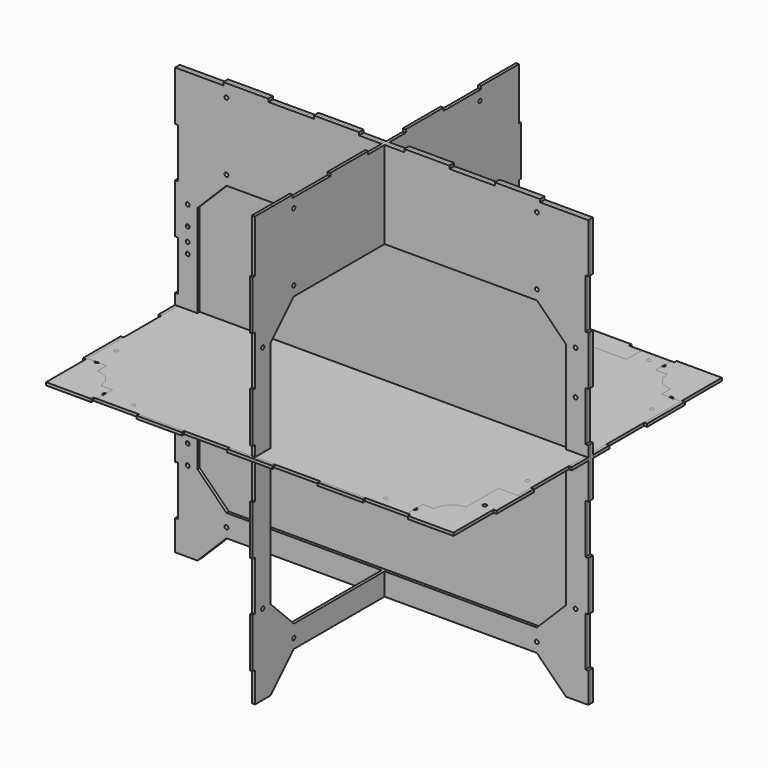
from build123d import *

# Parameters (mm, degrees)
F1_R     = 2
F2_DEPTH = 3
F3_R     = 2
F4_DEPTH = 3
F5_DEPTH = 3
F6_R     = 2
F7_DEPTH = 3
F8_R     = 2
F9_DEPTH = 3


# Not quite as in the source:
# - a feature names something its author has since deleted; it is built from what else it names


with BuildPart() as f2:
    # F1 (on Top) → F2 (new body)
    with BuildSketch(Plane.XY):
        Polygon((163.3333333333, -173), (210, -173), (210, -170), (210, -121.4285714286), (213, -121.4285714286), (213, -72.8571428571), (210, -72.8571428571), (210, -24.2857142857), (213, -24.2857142857), (213, 24.2857142857), (210, 24.2857142857), (210, 72.8571428571), (213, 72.8571428571), (213, 121.4285714286), (210, 121.4285714286), (210, 170), (210, 173), (163.3333333333, 173), (163.3333333333, 170), (116.6666666667, 170), (116.6666666667, 173), (70, 173), (70, 170), (23.3333333333, 170), (23.3333333333, 173), (-23.3333333333, 173), (-23.3333333333, 170), (-70, 170), (-70, 173), (-116.6666666667, 173), (-116.6666666667, 170), (-163.3333333333, 170), (-163.3333333333, 173), (-210, 173), (-210, 170), (-210, 121.4285714286), (-213, 121.4285714286), (-213, 72.8571428571), (-210, 72.8571428571), (-210, 24.2857142857), (-213, 24.2857142857), (-213, -24.2857142857), (-210, -24.2857142857), (-210, -72.8571428571), (-213, -72.8571428571), (-213, -121.4285714286), (-210, -121.4285714286), (-210, -170), (-210, -173), (-163.3333333333, -173), (-163.3333333333, -170), (-116.6666666667, -170), (-116.6666666667, -173), (-70, -173), (-70, -170), (-23.3333333333, -170), (-23.3333333333, -173), (23.3333333333, -173), (23.3333333333, -170), (70, -170), (70, -173), (116.6666666667, -173), (116.6666666667, -170), (163.3333333333, -170), align=None)
        with Locations((-160, -160)):
            Circle(F1_R, mode=Mode.SUBTRACT)
        with Locations((-200, -120)):
            Circle(F1_R, mode=Mode.SUBTRACT)
        with Locations((160, -160)):
            Circle(F1_R, mode=Mode.SUBTRACT)
        with Locations((200, -120)):
            Circle(F1_R, mode=Mode.SUBTRACT)
        with Locations((-200, 120)):
            Circle(F1_R, mode=Mode.SUBTRACT)
        with Locations((-160, 160)):
            Circle(F1_R, mode=Mode.SUBTRACT)
        Polygon((190, -120), (160, -150), (-160, -150), (-190, -120), (-190, 120), (-160, 150), (160, 150), (190, 120), align=None, mode=Mode.SUBTRACT)
        with Locations((200, 120)):
            Circle(F1_R, mode=Mode.SUBTRACT)
        with Locations((160, 160)):
            Circle(F1_R, mode=Mode.SUBTRACT)
    extrude(amount=F2_DEPTH)


with BuildPart() as f4:
    # F3 (on Front) → F4 (new body)
    with BuildSketch(Plane.XZ):
        Polygon((190, -221.5), (213, -221.5), (213, -190.3888888889), (210, -190.3888888889), (210, -139.2777777778), (213, -139.2777777778), (213, -88.1666666667), (210, -88.1666666667), (210, -37.0555555556), (213, -37.0555555556), (213, 14.0555555556), (210, 14.0555555556), (210, 65.1666666667), (213, 65.1666666667), (213, 116.2777777778), (210, 116.2777777778), (210, 167.3888888889), (213, 167.3888888889), (213, 218.5), (210, 218.5), (163.3333333333, 218.5), (163.3333333333, 221.5), (116.6666666667, 221.5), (116.6666666667, 218.5), (70, 218.5), (70, 221.5), (23.3333333333, 221.5), (23.3333333333, 218.5), (-23.3333333333, 218.5), (-23.3333333333, 221.5), (-70, 221.5), (-70, 218.5), (-116.6666666667, 218.5), (-116.6666666667, 221.5), (-163.3333333333, 221.5), (-163.3333333333, 218.5), (-210, 218.5), (-213, 218.5), (-213, 167.3888888889), (-210, 167.3888888889), (-210, 116.2777777778), (-213, 116.2777777778), (-213, 65.1666666667), (-210, 65.1666666667), (-210, 14.0555555556), (-213, 14.0555555556), (-213, -37.0555555556), (-210, -37.0555555556), (-210, -88.1666666667), (-213, -88.1666666667), (-213, -139.2777777778), (-210, -139.2777777778), (-210, -190.3888888889), (-213, -190.3888888889), (-213, -221.5), (-190, -221.5), (-160, -191.5), (160, -191.5), align=None)
        with Locations((-160, -181.5)):
            Circle(F3_R, mode=Mode.SUBTRACT)
        with Locations((-200, -138.5)):
            Circle(F3_R, mode=Mode.SUBTRACT)
        with Locations((-200, -118.5)):
            Circle(F3_R, mode=Mode.SUBTRACT)
        with Locations((-200, -104.5)):
            Circle(F3_R, mode=Mode.SUBTRACT)
        with Locations((160, -181.5)):
            Circle(F3_R, mode=Mode.SUBTRACT)
        with Locations((200, -138.5)):
            Circle(F3_R, mode=Mode.SUBTRACT)
        Polygon((-160, 128.5), (160, 128.5), (190, 98.5), (190, -138.5), (160, -168.5), (-160, -168.5), (-190, -138.5), (-190, 98.5), align=None, mode=Mode.SUBTRACT)
        with Locations((-200, 53.5)):
            Circle(F3_R, mode=Mode.SUBTRACT)
        with Locations((-200, 64.5)):
            Circle(F3_R, mode=Mode.SUBTRACT)
        with Locations((-200, 78.5)):
            Circle(F3_R, mode=Mode.SUBTRACT)
        with Locations((-200, 98.5)):
            Circle(F3_R, mode=Mode.SUBTRACT)
        with Locations((-160, 138.5)):
            Circle(F3_R, mode=Mode.SUBTRACT)
        with Locations((-160, 208.5)):
            Circle(F3_R, mode=Mode.SUBTRACT)
        with Locations((-140, 208.5)):
            Circle(F3_R, mode=Mode.SUBTRACT)
        with Locations((-126, 208.5)):
            Circle(F3_R, mode=Mode.SUBTRACT)
        with Locations((200, 53.5)):
            Circle(F3_R, mode=Mode.SUBTRACT)
        with Locations((200, 98.5)):
            Circle(F3_R, mode=Mode.SUBTRACT)
        with Locations((160, 138.5)):
            Circle(F3_R, mode=Mode.SUBTRACT)
        with Locations((126, 208.5)):
            Circle(F3_R, mode=Mode.SUBTRACT)
        with Locations((140, 208.5)):
            Circle(F3_R, mode=Mode.SUBTRACT)
        with Locations((160, 208.5)):
            Circle(F3_R, mode=Mode.SUBTRACT)
        with Locations((-140, 208.5)):
            Circle(F3_R)
        with Locations((-126, 208.5)):
            Circle(F3_R)
        with Locations((126, 208.5)):
            Circle(F3_R)
        with Locations((140, 208.5)):
            Circle(F3_R)
    extrude(amount=F4_DEPTH)


with BuildPart() as f5:
    # F3 (on Front) → F5 (new body)
    with BuildSketch(Plane.XZ):
        Polygon((190, -221.5), (213, -221.5), (213, -190.3888888889), (210, -190.3888888889), (210, -139.2777777778), (213, -139.2777777778), (213, -88.1666666667), (210, -88.1666666667), (210, -37.0555555556), (213, -37.0555555556), (213, 14.0555555556), (210, 14.0555555556), (210, 65.1666666667), (213, 65.1666666667), (213, 116.2777777778), (210, 116.2777777778), (210, 167.3888888889), (213, 167.3888888889), (213, 218.5), (210, 218.5), (163.3333333333, 218.5), (163.3333333333, 221.5), (116.6666666667, 221.5), (116.6666666667, 218.5), (70, 218.5), (70, 221.5), (23.3333333333, 221.5), (23.3333333333, 218.5), (-23.3333333333, 218.5), (-23.3333333333, 221.5), (-70, 221.5), (-70, 218.5), (-116.6666666667, 218.5), (-116.6666666667, 221.5), (-163.3333333333, 221.5), (-163.3333333333, 218.5), (-210, 218.5), (-213, 218.5), (-213, 167.3888888889), (-210, 167.3888888889), (-210, 116.2777777778), (-213, 116.2777777778), (-213, 65.1666666667), (-210, 65.1666666667), (-210, 14.0555555556), (-213, 14.0555555556), (-213, -37.0555555556), (-210, -37.0555555556), (-210, -88.1666666667), (-213, -88.1666666667), (-213, -139.2777777778), (-210, -139.2777777778), (-210, -190.3888888889), (-213, -190.3888888889), (-213, -221.5), (-190, -221.5), (-160, -191.5), (160, -191.5), align=None)
        with Locations((-160, -181.5)):
            Circle(F3_R, mode=Mode.SUBTRACT)
        with Locations((-200, -138.5)):
            Circle(F3_R, mode=Mode.SUBTRACT)
        with Locations((-200, -118.5)):
            Circle(F3_R, mode=Mode.SUBTRACT)
        with Locations((-200, -104.5)):
            Circle(F3_R, mode=Mode.SUBTRACT)
        with Locations((160, -181.5)):
            Circle(F3_R, mode=Mode.SUBTRACT)
        with Locations((200, -138.5)):
            Circle(F3_R, mode=Mode.SUBTRACT)
        Polygon((-160, 128.5), (160, 128.5), (190, 98.5), (190, -138.5), (160, -168.5), (-160, -168.5), (-190, -138.5), (-190, 98.5), align=None, mode=Mode.SUBTRACT)
        with Locations((-200, 53.5)):
            Circle(F3_R, mode=Mode.SUBTRACT)
        with Locations((-200, 64.5)):
            Circle(F3_R, mode=Mode.SUBTRACT)
        with Locations((-200, 78.5)):
            Circle(F3_R, mode=Mode.SUBTRACT)
        with Locations((-200, 98.5)):
            Circle(F3_R, mode=Mode.SUBTRACT)
        with Locations((-160, 138.5)):
            Circle(F3_R, mode=Mode.SUBTRACT)
        with Locations((-160, 208.5)):
            Circle(F3_R, mode=Mode.SUBTRACT)
        with Locations((-140, 208.5)):
            Circle(F3_R, mode=Mode.SUBTRACT)
        with Locations((-126, 208.5)):
            Circle(F3_R, mode=Mode.SUBTRACT)
        with Locations((200, 53.5)):
            Circle(F3_R, mode=Mode.SUBTRACT)
        with Locations((200, 98.5)):
            Circle(F3_R, mode=Mode.SUBTRACT)
        with Locations((160, 138.5)):
            Circle(F3_R, mode=Mode.SUBTRACT)
        with Locations((126, 208.5)):
            Circle(F3_R, mode=Mode.SUBTRACT)
        with Locations((140, 208.5)):
            Circle(F3_R, mode=Mode.SUBTRACT)
        with Locations((160, 208.5)):
            Circle(F3_R, mode=Mode.SUBTRACT)
        Polygon((190, 98.5), (160, 128.5), (-160, 128.5), (-190, 98.5), (-190, -138.5), (-160, -168.5), (160, -168.5), (190, -138.5), align=None)
        with BuildLine():
            Line((160, -15), (160, -10))
            ThreePointArc((160, -10), (170, -20), (160, -30))
            Line((160, -30), (160, -25))
            ThreePointArc((160, -25), (155, -20), (160, -15))
        make_face(mode=Mode.SUBTRACT)
        with Locations((-200, 78.5)):
            Circle(F3_R)
        with Locations((-200, -104.5)):
            Circle(F3_R)
        with Locations((-200, -118.5)):
            Circle(F3_R)
        with BuildLine():
            ThreePointArc((160, -30), (170, -20), (160, -10))
            Line((160, -10), (160, -15))
            ThreePointArc((160, -15), (155, -20), (160, -25))
            Line((160, -25), (160, -30))
        make_face()
    extrude(amount=-F5_DEPTH)


with BuildPart() as f7:
    # F6 (on Right) → F7 (new body)
    with BuildSketch(Plane.YZ):
        Polygon((-170, -221.5), (-150, -221.5), (-120, -191.5), (120, -191.5), (150, -221.5), (170, -221.5), (170, -190.3888888889), (173, -190.3888888889), (173, -139.2777777778), (170, -139.2777777778), (170, -88.1666666667), (173, -88.1666666667), (173, -37.0555555556), (170, -37.0555555556), (170, 14.0555555556), (173, 14.0555555556), (173, 65.1666666667), (170, 65.1666666667), (170, 116.2777777778), (173, 116.2777777778), (173, 167.3888888889), (170, 167.3888888889), (170, 218.5), (170, 221.5), (121.4285714286, 221.5), (121.4285714286, 218.5), (72.8571428571, 218.5), (72.8571428571, 221.5), (24.2857142857, 221.5), (24.2857142857, 218.5), (-24.2857142857, 218.5), (-24.2857142857, 221.5), (-72.8571428571, 221.5), (-72.8571428571, 218.5), (-121.4285714286, 218.5), (-121.4285714286, 221.5), (-170, 221.5), (-170, 218.5), (-170, 167.3888888889), (-173, 167.3888888889), (-173, 116.2777777778), (-170, 116.2777777778), (-170, 65.1666666667), (-173, 65.1666666667), (-173, 14.0555555556), (-170, 14.0555555556), (-170, -37.0555555556), (-173, -37.0555555556), (-173, -88.1666666667), (-170, -88.1666666667), (-170, -139.2777777778), (-173, -139.2777777778), (-173, -190.3888888889), (-170, -190.3888888889), align=None)
        with Locations((-120, -181.5)):
            Circle(F6_R, mode=Mode.SUBTRACT)
        with Locations((-160, -138.5)):
            Circle(F6_R, mode=Mode.SUBTRACT)
        with Locations((120, -181.5)):
            Circle(F6_R, mode=Mode.SUBTRACT)
        with Locations((160, -138.5)):
            Circle(F6_R, mode=Mode.SUBTRACT)
        with Locations((160, -118.5)):
            Circle(F6_R, mode=Mode.SUBTRACT)
        Polygon((-150, 98.5), (-120, 128.5), (120, 128.5), (150, 98.5), (150, -138.5), (120, -168.5), (-120, -168.5), (-150, -138.5), align=None, mode=Mode.SUBTRACT)
        with Locations((160, -104.5)):
            Circle(F6_R, mode=Mode.SUBTRACT)
        with Locations((-160, 98.5)):
            Circle(F6_R, mode=Mode.SUBTRACT)
        with Locations((-120, 138.5)):
            Circle(F6_R, mode=Mode.SUBTRACT)
        with Locations((-120, 208.5)):
            Circle(F6_R, mode=Mode.SUBTRACT)
        with Locations((160, 64.5)):
            Circle(F6_R, mode=Mode.SUBTRACT)
        with Locations((160, 78.5)):
            Circle(F6_R, mode=Mode.SUBTRACT)
        with Locations((160, 98.5)):
            Circle(F6_R, mode=Mode.SUBTRACT)
        with Locations((120, 138.5)):
            Circle(F6_R, mode=Mode.SUBTRACT)
        with Locations((120, 208.5)):
            Circle(F6_R, mode=Mode.SUBTRACT)
    extrude(amount=F7_DEPTH)


with BuildPart() as f9:
    # F8 (on Top) → F9 (new body)
    with BuildSketch(Plane.XY):
        with BuildLine():
            Line((160, -150), (172, -150))
            ThreePointArc((172, -150), (177.2720779386, -137.2720779386), (190, -132))
            Line((190, -132), (190, -90))
            Line((190, -90), (210, -90))
            Line((210, -90), (210, 120))
            Line((210, 120), (190, 120))
            Line((190, 120), (190, 132))
            ThreePointArc((190, 132), (177.2720779386, 137.2720779386), (172, 150))
            Line((172, 150), (160, 150))
            Line((160, 150), (160, 170))
            Line((160, 170), (130, 170))
            Line((130, 170), (130, 150))
            Line((130, 150), (37.5, 150))
            Line((37.5, 150), (37.5, 147))
            Line((37.5, 147), (24.5, 147))
            Line((24.5, 147), (24.5, 107))
            Line((24.5, 107), (-24.5, 107))
            Line((-24.5, 107), (-24.5, 147))
            Line((-24.5, 147), (-37.5, 147))
            Line((-37.5, 147), (-37.5, 150))
            Line((-37.5, 150), (-130, 150))
            Line((-130, 150), (-130, 170))
            Line((-130, 170), (-160, 170))
            Line((-160, 170), (-160, 150))
            Line((-160, 150), (-172, 150))
            ThreePointArc((-172, 150), (-177.2720779386, 137.2720779386), (-190, 132))
            Line((-190, 132), (-190, 90))
            Line((-190, 90), (-210, 90))
            Line((-210, 90), (-210, -120))
            Line((-210, -120), (-190, -120))
            Line((-190, -120), (-190, -132))
            ThreePointArc((-190, -132), (-177.2720779386, -137.2720779386), (-172, -150))
            Line((-172, -150), (-160, -150))
            Line((-160, -150), (-160, -170))
            Line((-160, -170), (160, -170))
            Line((160, -170), (160, -150))
        make_face()
        with Locations((-130, -160)):
            Circle(F8_R, mode=Mode.SUBTRACT)
        with Locations((-200, -95)):
            Circle(F8_R, mode=Mode.SUBTRACT)
        with Locations((130, -160)):
            Circle(F8_R, mode=Mode.SUBTRACT)
        with Locations((200, -65)):
            Circle(F8_R, mode=Mode.SUBTRACT)
        with Locations((-200, 65)):
            Circle(F8_R, mode=Mode.SUBTRACT)
        with Locations((-145, 160)):
            Circle(F8_R, mode=Mode.SUBTRACT)
        with Locations((200, 95)):
            Circle(F8_R, mode=Mode.SUBTRACT)
        with Locations((145, 160)):
            Circle(F8_R, mode=Mode.SUBTRACT)
    extrude(amount=F9_DEPTH)


solid = Compound([f2.part, f4.part, f5.part, f7.part, f9.part])
